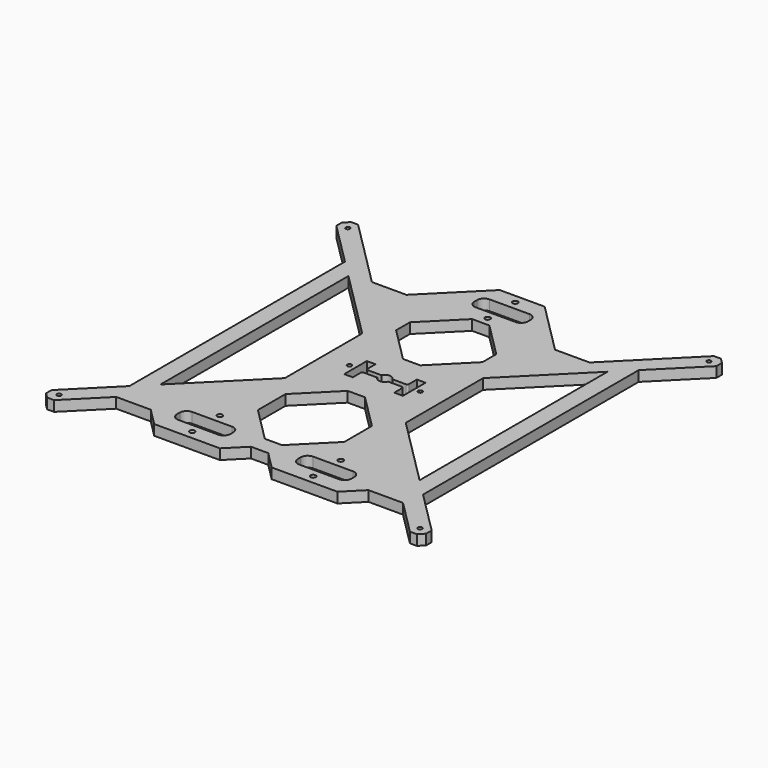
from build123d import *

# Parameters (mm, degrees)
F0_R     = 1.2295
F0_R_2   = 1.5
F1_DEPTH = 6


# Not quite as in the source:
# - ends of sketch curves that miss each other by under 0.0002 mm in the source are joined


with BuildPart() as f1:
    # F0 (on Top) → F1 (new body)
    with BuildSketch(Plane.XY):
        Polygon((-110, -103), (-110, -107), (-107, -110), (-103, -110), (-83, -90), (-63, -90), (-53, -100), (-15, -100), (-5, -90), (5, -90), (15, -100), (53, -100), (63, -90), (83, -90), (103, -110), (107, -110), (110, -107), (110, -103), (85, -78), (85, 78), (110, 103), (110, 107), (107, 110), (103, 110), (63, 70), (43, 70), (13, 100), (-13, 100), (-43, 70), (-63, 70), (-103, 110), (-107, 110), (-110, 107), (-110, 103), (-85, 78), (-85, -78), align=None)
        with Locations((-104.5, -104.5)):
            Circle(F0_R, mode=Mode.SUBTRACT)
        with Locations((-34.999989, -95.000012)):
            Circle(F0_R_2, mode=Mode.SUBTRACT)
        with BuildLine():
            ThreePointArc((-20.007037, -86), (-21.1786098753, -88.8284271247), (-24.007037, -90))
            Line((-24.007037, -90), (-47.007037, -90))
            ThreePointArc((-47.007037, -90), (-49.8354641247, -88.8284271247), (-51.007037, -86))
            Line((-51.007037, -86), (-51.007037, -84))
            ThreePointArc((-51.007037, -84), (-49.8354641247, -81.1715728753), (-47.007037, -80))
            Line((-47.007037, -80), (-24.007037, -80))
            ThreePointArc((-24.007037, -80), (-21.1786098753, -81.1715728753), (-20.007037, -84))
            Line((-20.007037, -84), (-20.007037, -86))
        make_face(mode=Mode.SUBTRACT)
        with Locations((-34.999989, -75.000012)):
            Circle(F0_R_2, mode=Mode.SUBTRACT)
        with Locations((35.000011, -95.000012)):
            Circle(F0_R_2, mode=Mode.SUBTRACT)
        with BuildLine():
            ThreePointArc((50, -86), (48.8284271247, -88.8284271247), (46, -90))
            Line((46, -90), (23, -90))
            ThreePointArc((23, -90), (20.1715728753, -88.8284271247), (19, -86))
            Line((19, -86), (19, -84))
            ThreePointArc((19, -84), (20.1715728753, -81.1715728753), (23, -80))
            Line((23, -80), (46, -80))
            ThreePointArc((46, -80), (48.8284271247, -81.1715728753), (50, -84))
            Line((50, -84), (50, -86))
        make_face(mode=Mode.SUBTRACT)
        with Locations((35.000011, -75.000012)):
            Circle(F0_R_2, mode=Mode.SUBTRACT)
        with Locations((104.5, -104.5)):
            Circle(F0_R, mode=Mode.SUBTRACT)
        Polygon((25, -60), (5, -80), (-5, -80), (-25, -60), (-25, -40), (-5, -20), (5, -20), (25, -40), align=None, mode=Mode.SUBTRACT)
        Polygon((-75, -68), (-75, 68), (-35, 28), (-35, -28), align=None, mode=Mode.SUBTRACT)
        with Locations((-20, 0)):
            Circle(F0_R, mode=Mode.SUBTRACT)
        with Locations((-104.5, 104.5)):
            Circle(F0_R, mode=Mode.SUBTRACT)
        with BuildLine():
            Line((-16.5, -8.2), (-16.5, 8.2))
            Line((-16.5, 8.2), (-11.5, 8.2))
            Line((-11.5, 8.2), (-11.5, 2.5))
            ThreePointArc((-11.5, 2.5), (-11.2071067812, 1.7928932188), (-10.5, 1.5))
            Line((-10.5, 1.5), (-2.662278, 1.5))
            ThreePointArc((-2.662278, 1.5), (0.4999997857, 3.5), (3.6622775389, 1.5000002556))
            Line((3.6622775389, 1.5000002556), (11.5, 1.5))
            ThreePointArc((11.5, 1.5), (12.2071067812, 1.7928932188), (12.5, 2.5))
            Line((12.5, 2.5), (12.5, 8.2))
            Line((12.5, 8.2), (17.5, 8.2))
            Line((17.5, 8.2), (17.5, -8.2))
            Line((17.5, -8.2), (12.5, -8.2))
            Line((12.5, -8.2), (12.5, -2.5))
            ThreePointArc((12.5, -2.5), (12.2071067812, -1.7928932188), (11.5, -1.5))
            Line((11.5, -1.5), (3.662277, -1.5))
            ThreePointArc((3.662277, -1.5), (0.4999997857, -3.5), (-2.6622777226, -1.4999998684))
            Line((-2.6622777226, -1.4999998684), (-10.5, -1.5))
            ThreePointArc((-10.5, -1.5), (-11.2071067812, -1.7928932188), (-11.5, -2.5))
            Line((-11.5, -2.5), (-11.5, -8.2))
            Line((-11.5, -8.2), (-16.5, -8.2))
        make_face(mode=Mode.SUBTRACT)
        with Locations((21, 0)):
            Circle(F0_R, mode=Mode.SUBTRACT)
        Polygon((-5, 20), (-25, 40), (-25, 50), (-5, 70), (5, 70), (25, 50), (25, 40), (5, 20), align=None, mode=Mode.SUBTRACT)
        Polygon((75, 68), (75, -68), (35, -28), (35, 28), align=None, mode=Mode.SUBTRACT)
        with Locations((1.1e-05, 74.999988)):
            Circle(F0_R_2, mode=Mode.SUBTRACT)
        with BuildLine():
            ThreePointArc((16.137123, 84), (14.9655501247, 81.1715728753), (12.137123, 80))
            Line((12.137123, 80), (-10.862877, 80))
            ThreePointArc((-10.862877, 80), (-13.6913041247, 81.1715728753), (-14.862877, 84))
            Line((-14.862877, 84), (-14.862877, 86))
            ThreePointArc((-14.862877, 86), (-13.6913041247, 88.8284271247), (-10.862877, 90))
            Line((-10.862877, 90), (12.137123, 90))
            ThreePointArc((12.137123, 90), (14.9655501247, 88.8284271247), (16.137123, 86))
            Line((16.137123, 86), (16.137123, 84))
        make_face(mode=Mode.SUBTRACT)
        with Locations((1.1e-05, 94.999988)):
            Circle(F0_R_2, mode=Mode.SUBTRACT)
        with Locations((104.5, 104.5)):
            Circle(F0_R, mode=Mode.SUBTRACT)
    extrude(amount=F1_DEPTH)


solid = f1.part
